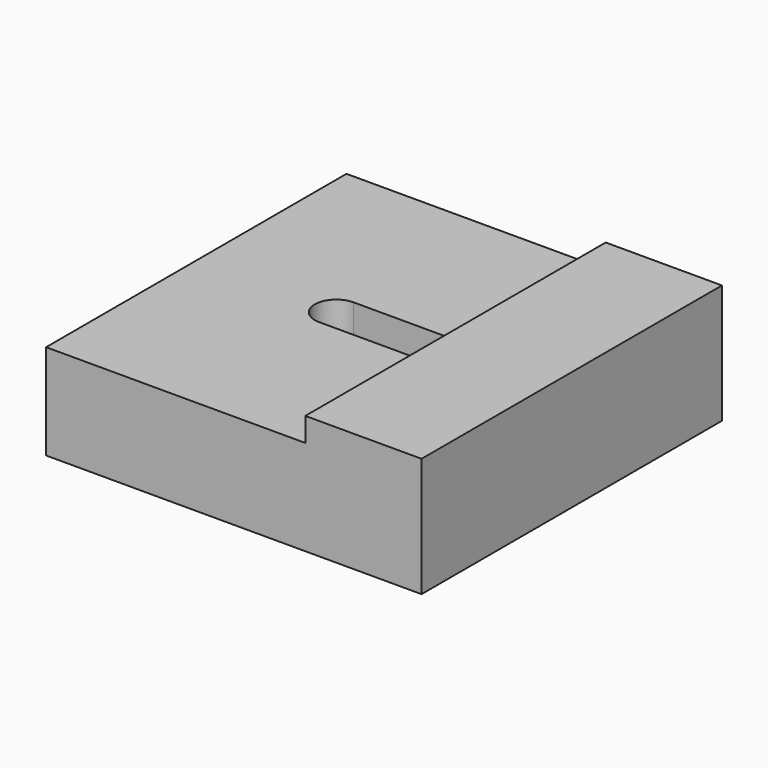
from build123d import *

# Parameters (mm, degrees)
F0_W     = 27.6225
F0_H     = 40.005
F0_R     = 3.302
F0_W_2   = 12.3825
F0_R_2   = 2.159
F1_DEPTH = 10.16
F2_DEPTH = 12.7
F4_DEPTH = 25.4
F5_DEPTH = 5.08
F6_DEPTH = 12.7
F8_D     = 2.9464
F8_DEPTH = 7.62
F8_TIP   = 0.885187864


# Not quite as in the source:
# - a feature names something its author has since deleted; it is built from what else it names


with BuildPart() as f1:
    # F0 (on Top) → F1 (new body)
    with BuildSketch(Plane.XY):
        with Locations((-6.19125, 0)):
            Rectangle(F0_W, F0_H)
        with Locations((-15.875, -15.875)):
            Circle(F0_R, mode=Mode.SUBTRACT)
        with Locations((-15.875, 15.875)):
            Circle(F0_R, mode=Mode.SUBTRACT)
        with Locations((13.81125, 0)):
            Rectangle(F0_W_2, F0_H)
        with Locations((15.875, -15.875)):
            Circle(F0_R, mode=Mode.SUBTRACT)
        with Locations((15.875, 15.875)):
            Circle(F0_R, mode=Mode.SUBTRACT)
        with Locations((-15.875, 15.875)):
            Circle(F0_R)
        with Locations((-15.875, 15.875)):
            Circle(F0_R_2, mode=Mode.SUBTRACT)
        with Locations((15.875, 15.875)):
            Circle(F0_R)
        with Locations((15.875, 15.875)):
            Circle(F0_R_2, mode=Mode.SUBTRACT)
        with Locations((15.875, -15.875)):
            Circle(F0_R)
        with Locations((15.875, -15.875)):
            Circle(F0_R_2, mode=Mode.SUBTRACT)
        with Locations((-15.875, -15.875)):
            Circle(F0_R)
        with Locations((-15.875, -15.875)):
            Circle(F0_R_2, mode=Mode.SUBTRACT)
        with Locations((-15.875, 15.875)):
            Circle(F0_R_2)
        with Locations((15.875, 15.875)):
            Circle(F0_R_2)
        with Locations((15.875, -15.875)):
            Circle(F0_R_2)
        with Locations((-15.875, -15.875)):
            Circle(F0_R_2)
    extrude(amount=F1_DEPTH)

    # F0 (on Top) → F2 (join)
    with BuildSketch(Plane.XY):
        with Locations((13.81125, 0)):
            Rectangle(F0_W_2, F0_H)
        with Locations((15.875, -15.875)):
            Circle(F0_R, mode=Mode.SUBTRACT)
        with Locations((15.875, 15.875)):
            Circle(F0_R, mode=Mode.SUBTRACT)
    extrude(amount=F2_DEPTH)

    # F3 (on face) → F4 (cut)
    with BuildSketch(Plane(origin=(0, 0, 0), x_dir=(1, 0, 0), z_dir=(0, 0, -1))):
        with BuildLine():
            ThreePointArc((-2.794, 0), (-3.4635538982, 1.6164461018), (-5.08, 2.286))
            ThreePointArc((-5.08, 2.286), (-7.366, 0), (-5.08, -2.286))
            ThreePointArc((-5.08, -2.286), (-3.4635538982, -1.6164461018), (-2.794, 0))
        make_face()
        with BuildLine():
            ThreePointArc((7.366, 0), (6.6964461018, 1.6164461018), (5.08, 2.286))
            ThreePointArc((5.08, 2.286), (2.794, 0), (5.08, -2.286))
            ThreePointArc((5.08, -2.286), (6.6964461018, -1.6164461018), (7.366, 0))
        make_face()
        with BuildLine():
            ThreePointArc((-1.27, 0), (-1.4655166344, 1.2048277885), (-2.032, 2.286))
            Line((-2.032, 2.286), (-5.08, 2.286))
            ThreePointArc((-5.08, 2.286), (-3.4635538982, 1.6164461018), (-2.794, 0))
            ThreePointArc((-2.794, 0), (-3.4635538982, -1.6164461018), (-5.08, -2.286))
            Line((-5.08, -2.286), (-2.032, -2.286))
            ThreePointArc((-2.032, -2.286), (-1.4655166344, -1.2048277885), (-1.27, 0))
        make_face()
        with BuildLine():
            ThreePointArc((2.032, -2.286), (1.27, 0), (2.032, 2.286))
            Line((2.032, 2.286), (-2.032, 2.286))
            ThreePointArc((-2.032, 2.286), (-1.4655166344, 1.2048277885), (-1.27, 0))
            ThreePointArc((-1.27, 0), (-1.4655166344, -1.2048277885), (-2.032, -2.286))
            Line((-2.032, -2.286), (2.032, -2.286))
        make_face()
        with BuildLine():
            Line((5.08, 2.286), (2.032, 2.286))
            ThreePointArc((2.032, 2.286), (1.27, 0), (2.032, -2.286))
            Line((2.032, -2.286), (5.08, -2.286))
            ThreePointArc((5.08, -2.286), (2.794, 0), (5.08, 2.286))
        make_face()
    extrude(amount=-F4_DEPTH, mode=Mode.SUBTRACT)

    # F3 (on face) → F5 (cut)
    with BuildSketch(Plane(origin=(0, 0, 0), x_dir=(1, 0, 0), z_dir=(0, 0, -1))):
        with BuildLine():
            ThreePointArc((-1.27, 0), (-1.4655166344, 1.2048277885), (-2.032, 2.286))
            Line((-2.032, 2.286), (-5.08, 2.286))
            ThreePointArc((-5.08, 2.286), (-3.4635538982, 1.6164461018), (-2.794, 0))
            ThreePointArc((-2.794, 0), (-3.4635538982, -1.6164461018), (-5.08, -2.286))
            Line((-5.08, -2.286), (-2.032, -2.286))
            ThreePointArc((-2.032, -2.286), (-1.4655166344, -1.2048277885), (-1.27, 0))
        make_face()
        with BuildLine():
            ThreePointArc((-2.032, 2.286), (-3.3761162011, 3.4077675977), (-5.08, 3.81))
            ThreePointArc((-5.08, 3.81), (-8.89, 0), (-5.08, -3.81))
            ThreePointArc((-5.08, -3.81), (-3.3761162011, -3.4077675977), (-2.032, -2.286))
            Line((-2.032, -2.286), (-5.08, -2.286))
            ThreePointArc((-5.08, -2.286), (-7.366, 0), (-5.08, 2.286))
            Line((-5.08, 2.286), (-2.032, 2.286))
        make_face()
        with BuildLine():
            ThreePointArc((2.032, 2.286), (3.3761162011, 3.4077675977), (5.08, 3.81))
            Line((5.08, 3.81), (-5.08, 3.81))
            ThreePointArc((-5.08, 3.81), (-3.3761162011, 3.4077675977), (-2.032, 2.286))
            Line((-2.032, 2.286), (2.032, 2.286))
        make_face()
        with BuildLine():
            ThreePointArc((2.032, -2.286), (1.27, 0), (2.032, 2.286))
            Line((2.032, 2.286), (-2.032, 2.286))
            ThreePointArc((-2.032, 2.286), (-1.4655166344, 1.2048277885), (-1.27, 0))
            ThreePointArc((-1.27, 0), (-1.4655166344, -1.2048277885), (-2.032, -2.286))
            Line((-2.032, -2.286), (2.032, -2.286))
        make_face()
        with BuildLine():
            Line((5.08, 2.286), (2.032, 2.286))
            ThreePointArc((2.032, 2.286), (1.27, 0), (2.032, -2.286))
            Line((2.032, -2.286), (5.08, -2.286))
            ThreePointArc((5.08, -2.286), (2.794, 0), (5.08, 2.286))
        make_face()
        with BuildLine():
            ThreePointArc((5.08, -3.81), (7.7740768363, -2.6940768363), (8.89, 0))
            ThreePointArc((8.89, 0), (7.7740768363, 2.6940768363), (5.08, 3.81))
            ThreePointArc((5.08, 3.81), (3.3761162011, 3.4077675977), (2.032, 2.286))
            Line((2.032, 2.286), (5.08, 2.286))
            ThreePointArc((5.08, 2.286), (6.6964461018, 1.6164461018), (7.366, 0))
            ThreePointArc((7.366, 0), (6.6964461018, -1.6164461018), (5.08, -2.286))
            Line((5.08, -2.286), (2.032, -2.286))
            ThreePointArc((2.032, -2.286), (3.3761162011, -3.4077675977), (5.08, -3.81))
        make_face()
        with BuildLine():
            Line((-5.08, -3.81), (5.08, -3.81))
            ThreePointArc((5.08, -3.81), (3.3761162011, -3.4077675977), (2.032, -2.286))
            Line((2.032, -2.286), (-2.032, -2.286))
            ThreePointArc((-2.032, -2.286), (-3.3761162011, -3.4077675977), (-5.08, -3.81))
        make_face()
    extrude(amount=-F5_DEPTH, mode=Mode.SUBTRACT)

    # F0 (on Top) → F6 (join)
    with BuildSketch(Plane.XY):
        with Locations((15.875, 15.875)):
            Circle(F0_R)
        with Locations((15.875, 15.875)):
            Circle(F0_R_2, mode=Mode.SUBTRACT)
        with Locations((15.875, 15.875)):
            Circle(F0_R_2)
        with Locations((15.875, -15.875)):
            Circle(F0_R)
        with Locations((15.875, -15.875)):
            Circle(F0_R_2, mode=Mode.SUBTRACT)
        with Locations((15.875, -15.875)):
            Circle(F0_R_2)
    extrude(amount=F6_DEPTH)

    # F8
    with Locations(Plane(origin=(0, 0, 0), x_dir=(1, 0, 0), z_dir=(0, 0, -1))):
        with Locations((-15.87754, 15.87754), (15.87754, 15.87754), (15.87754, -15.87754), (-15.87754, -15.87754)):
            Hole(F8_D / 2, depth=F8_DEPTH)
            with Locations((0, 0, -(F8_DEPTH + F8_TIP / 2))):  # 118° drill point
                Cone(0, F8_D / 2, F8_TIP, mode=Mode.SUBTRACT)


solid = f1.part
